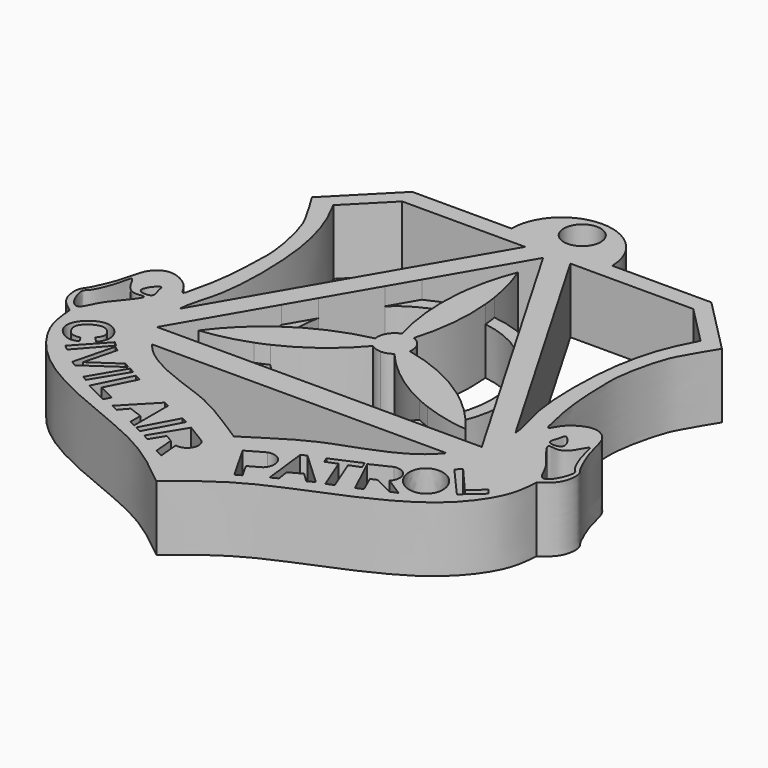
from build123d import *

# Parameters (mm, degrees)
F0_R     = 1.5875
F1_DEPTH = 5.588
F2_DEPTH = 4.064
F3_DEPTH = 3.175


# Not quite as in the source:
# - a feature names something its author has since deleted; it is built from what else it names


with BuildPart() as f1:
    # F0 (on Top) → F1 (new body)
    with BuildSketch(Plane.XY):
        with BuildLine():
            ThreePointArc((1.738595906, 17.4896921962), (-2.5962884327, 21.824576535), (-6.9311727715, 17.4896921962))
            Line((-6.9311727715, 17.4896921962), (-15.476684086, 17.4896921962))
            Line((-15.476684086, 17.4896921962), (-20.2500969172, 12.6594556496))
            add(Edge.make_bspline(
                [(-22.6898547262, -10.3722466156), (-23.0970195829, -10.0682558569), (-23.862899119, -9.4964474176), (-24.2116889935, -8.3793859815), (-24.1797927192, -7.4833620854), (-23.738938243, -7.0124281569), (-23.2773297932, -5.9756059833), (-22.8294147231, -4.8854228515), (-22.4842865284, -3.5101260949), (-22.2879650606, -2.7714005659), (-21.9081479252, -2.2626732598), (-21.271972846, -1.8143509905), (-20.3511303126, -1.7956869786), (-19.3559115764, -2.3311813439), (-18.720531189, -2.9569361713), (-18.2911432737, -3.9859192577), (-17.9733302285, -2.4199718419), (-17.4938217649, -0.258092059), (-17.3537315193, 2.707514965), (-17.2521862787, 5.0646604239), (-17.917211776, 8.1859371777), (-18.5482369005, 9.8853578959), (-19.692680388, 11.7416582003), (-20.0868858944, 12.3907254406), (-20.2500969172, 12.6594556496)],
                knots=[0, 0, 0, 0, 0.0480827662, 0.0904439714, 0.126688888, 0.1578769623, 0.1996629909, 0.244212497, 0.2916151482, 0.3262361378, 0.3571804574, 0.3915040257, 0.4288764076, 0.4706624253, 0.5103147505, 0.5426193777, 0.5825583957, 0.6451095501, 0.7133572635, 0.7758419326, 0.8458928164, 0.9011071458, 0.959055864, 1, 1, 1, 1], degree=3))
            add(Edge.make_bspline(
                [(-2.5962884327, -26.1529348791), (-3.3769549013, -25.509416408), (-4.9803315106, -24.1877220537), (-7.8461594134, -22.3308731385), (-12.0547247491, -20.6465778064), (-16.3768178003, -18.799451716), (-20.0336907945, -16.49456596), (-22.4832928257, -13.0808956511), (-22.6260637565, -11.2087384767), (-22.6898547262, -10.3722466156)],
                knots=[0, 0, 0, 0, 0.1283905799, 0.2636957792, 0.4203835822, 0.5806441644, 0.7340153977, 0.8811563698, 1, 1, 1, 1], degree=3))
            add(Edge.make_bspline(
                [(-2.5962884327, -26.1529348791), (-1.8156219642, -25.509416408), (-0.2122453549, -24.1877220537), (2.6535825479, -22.3308731385), (6.8621478837, -20.6465778064), (11.1842409349, -18.799451716), (14.841113929, -16.49456596), (17.2907159602, -13.0808956511), (17.433486891, -11.2087384767), (17.4972778607, -10.3722466156)],
                knots=[0, 0, 0, 0, 0.1283905799, 0.2636957792, 0.4203835822, 0.5806441644, 0.7340153977, 0.8811563698, 1, 1, 1, 1], degree=3))
            add(Edge.make_bspline(
                [(17.4972778607, -10.3722466156), (17.9044427174, -10.0682558569), (18.6703222535, -9.4964474176), (19.0191121281, -8.3793859815), (18.9872158537, -7.4833620854), (18.5463613775, -7.0124281569), (18.0847529277, -5.9756059833), (17.6368378576, -4.8854228515), (17.2917096629, -3.5101260949), (17.0953881952, -2.7714005659), (16.7155710597, -2.2626732598), (16.0793959805, -1.8143509905), (15.1585534472, -1.7956869786), (14.163334711, -2.3311813439), (13.5279543235, -2.9569361713), (13.0985664083, -3.9859192577), (12.780753363, -2.4199718419), (12.3012448994, -0.258092059), (12.1611546538, 2.707514965), (12.0596094132, 5.0646604239), (12.7246349105, 8.1859371777), (13.355660035, 9.8853578959), (14.5001035226, 11.7416582003), (14.8943090289, 12.3907254406), (15.0575200517, 12.6594556496)],
                knots=[0, 0, 0, 0, 0.0480827662, 0.0904439714, 0.126688888, 0.1578769623, 0.1996629909, 0.244212497, 0.2916151482, 0.3262361378, 0.3571804574, 0.3915040257, 0.4288764076, 0.4706624253, 0.5103147505, 0.5426193777, 0.5825583957, 0.6451095501, 0.7133572635, 0.7758419326, 0.8458928164, 0.9011071458, 0.959055864, 1, 1, 1, 1], degree=3))
            Line((15.0575200517, 12.6594556496), (10.2841072205, 17.4896921962))
            Line((10.2841072205, 17.4896921962), (1.738595906, 17.4896921962))
        make_face()
        Polygon((-17.8642552346, -16.1066018045), (-16.9762261212, -12.5996377319), (-16.5397357196, -12.9157155752), (-17.2622017562, -15.7002154738), (-14.9141903967, -14.089721255), (-14.4475987181, -14.3606457859), (-17.4127146602, -16.407629475), align=None, mode=Mode.SUBTRACT)
        Polygon((-15.9211166715, -17.3533935501), (-14.2067773268, -14.4359013066), (-13.7401847169, -14.7218769416), (-15.5081700509, -17.6064894405), align=None, mode=Mode.SUBTRACT)
        Polygon((-14.7967901412, -18.0994002604), (-13.2585410029, -15.0078516454), (-12.7166928723, -15.278775245), (-13.977994685, -17.801383206), (-12.5511270844, -18.51481578), (-12.8340924241, -19.0807474322), align=None, mode=Mode.SUBTRACT)
        with BuildLine():
            Line((-7.37993652, -21.467037499), (-5.6344987825, -18.6040941626))
            Line((-5.6344987825, -18.6040941626), (-3.8670410245, -19.6816521537))
            ThreePointArc((-3.8670410245, -19.6816521537), (-3.764117873, -20.8257670053), (-4.8256372102, -21.264821291))
            Line((-4.8256372102, -21.264821291), (-4.6681218682, -23.0358021975))
            Line((-4.6681218682, -23.0358021975), (-5.3577828221, -22.6909723133))
            Line((-5.3577828221, -22.6909723133), (-5.5061231892, -20.9627524731))
            Line((-5.5061231892, -20.9627524731), (-6.1475215606, -20.5717140239))
            Line((-6.1475215606, -20.5717140239), (-6.8794107919, -21.7721907597))
            Line((-6.8794107919, -21.7721907597), (-7.37993652, -21.467037499))
        make_face(mode=Mode.SUBTRACT)
        Polygon((-11.7684574798, -19.4329470396), (-9.2849843204, -16.8591663241), (-8.8304335127, -17.1150397509), (-8.8304335127, -20.7514461295), (-9.3602407724, -20.486542955), (-9.3602407724, -19.4178968668), (-10.5342464522, -18.9814064652), (-11.1784443342, -19.7279531053), align=None, mode=Mode.SUBTRACT)
        Polygon((-8.5421427919, -20.8859350641), (-6.9435769692, -17.9123040289), (-6.4029168751, -18.1826336113), (-7.9972250387, -21.1583934724), align=None, mode=Mode.SUBTRACT)
        with BuildLine():
            Line((-18.4221062809, -12.8449834883), (-18.8736468554, -12.3934429139))
            add(Edge.make_bspline(
                [(-19.6262151003, -13.0210751668), (-19.8367266487, -13.0430759324), (-20.3227133654, -13.1137191828), (-20.8027190675, -12.6674579998), (-21.1008981102, -11.9005360544), (-20.5338553761, -11.2320232518), (-19.6483014218, -10.7265798158), (-18.8566799506, -10.9897330227), (-18.4070316189, -11.7820741099), (-18.7210894211, -12.193564562), (-18.8736468554, -12.3934429139)],
                knots=[0, 0, 0, 0, 0.1176639127, 0.2306398841, 0.3539001056, 0.4832941963, 0.6263662227, 0.7518807406, 0.8786495407, 1, 1, 1, 1], degree=3))
            Line((-19.6262151003, -13.0210751668), (-19.3552915007, -13.4771401063))
            add(Edge.make_bspline(
                [(-19.3552915007, -13.4771401063), (-19.6647479685, -13.6277405765), (-20.2558959615, -13.7459268657), (-21.4140601271, -12.9898777242), (-21.7138181634, -11.531227757), (-20.0020523703, -10.0337422831), (-18.4976057776, -10.5493501512), (-17.8424780807, -11.8252496322), (-18.1724769863, -12.5210379384), (-18.4221062809, -12.8449834883)],
                knots=[0, 0, 0, 0, 0.1194322555, 0.2593120389, 0.401976621, 0.5782160681, 0.7265712091, 0.8676998255, 1, 1, 1, 1], degree=3))
        make_face(mode=Mode.SUBTRACT)
        Polygon((-19.6901927204, -14.5726281785), (-17.4127146602, -12.1029438451), (-17.0364305377, -12.4340727925), (-19.2552052424, -14.9554159103), align=None, mode=Mode.SUBTRACT)
        with BuildLine():
            add(Edge.make_bspline(
                [(-22.2999965351, -4.1639455594), (-22.1639318726, -4.1828168323), (-21.7194415576, -5.282103379), (-20.8572790048, -5.8501067699), (-19.5835447922, -5.4389447995), (-20.9052955663, -7.0779233036), (-21.9130983435, -8.2734402986), (-22.4890245815, -9.8966926591), (-23.4408419776, -9.1820975684), (-23.9767448866, -7.5276575791), (-23.4119779874, -7.3423168433), (-22.5552081146, -5.3265047979), (-22.4311477981, -4.1457557427), (-22.2999965351, -4.1639455594)],
                knots=[0, 0, 0, 0, 0.0883353731, 0.1758724355, 0.2462255334, 0.3448161859, 0.4603143006, 0.5549763071, 0.6307679108, 0.734848778, 0.7893482102, 0.9148544851, 1, 1, 1, 1], degree=3))
        make_face(mode=Mode.SUBTRACT)
        with BuildLine():
            add(Edge.make_bspline(
                [(-19.8393442792, -4.3678420189), (-19.7555659682, -4.7033214852), (-19.3308745145, -5.4325501492), (-21.474675776, -5.3829622431), (-19.8854959132, -3.4280208948), (-19.9054119199, -4.1032826531), (-19.8393442792, -4.3678420189)],
                knots=[0, 0, 0, 0, 0.2397998485, 0.5036254155, 0.8108936546, 1, 1, 1, 1], degree=3))
        make_face(mode=Mode.SUBTRACT)
        with BuildLine():
            Line((1.4085588329, -21.8684608151), (0.9114956483, -22.1504680812))
            Line((0.9114956483, -22.1504680812), (-0.8477756055, -19.0495941788))
            Line((-0.8477756055, -19.0495941788), (0.6198497044, -18.2169414814))
            ThreePointArc((0.6198497044, -18.2169414814), (1.9215311054, -18.7052821537), (1.7703687569, -20.0873100211))
            Line((1.7703687569, -20.0873100211), (0.7321975794, -20.6763132397))
            Line((0.7321975794, -20.6763132397), (1.4085588329, -21.8684608151))
        make_face(mode=Mode.SUBTRACT)
        Polygon((3.0251524877, -20.9860596806), (2.5695136283, -17.1257872134), (3.0124958139, -16.8979670852), (5.860236939, -19.5558592677), (5.3033456206, -19.8849327862), (4.4933212921, -19.100220874), (3.4428210929, -19.6697693318), (3.5947004799, -20.6949561834), align=None, mode=Mode.SUBTRACT)
        Polygon((4.4553512707, -16.8979670852), (4.2655020952, -16.4170153439), (6.7074126392, -15.3441904525), (6.9369611313, -15.9257138997), (6.0251991727, -16.2856195643), (7.1409758349, -19.1122566943), (6.5159392383, -19.3589814118), (5.3976596864, -16.5260036211), align=None, mode=Mode.SUBTRACT)
        with BuildLine():
            Line((8.4675019607, -18.593955785), (6.923393812, -15.3538584709))
            Line((6.923393812, -15.3538584709), (8.5989612084, -14.5553462599))
            ThreePointArc((8.5989612084, -14.5553462599), (9.7586835256, -15.0510769239), (9.6065988764, -16.3031052798))
            Line((9.6065988764, -16.3031052798), (11.1975504045, -17.3254568012))
            Line((11.1975504045, -17.3254568012), (10.5811590329, -17.5687689334))
            Line((10.5811590329, -17.5687689334), (8.9304475494, -16.7119012066))
            Line((8.9304475494, -16.7119012066), (8.4149169811, -16.9410266529))
            Line((8.4149169811, -16.9410266529), (9.0370504186, -18.3408223093))
            Line((9.0370504186, -18.3408223093), (8.4675019607, -18.593955785))
        make_face(mode=Mode.SUBTRACT)
        with BuildLine():
            add(Edge.make_bspline(
                [(10.3659965098, -13.3920814842), (8.3039293696, -15.1227450253), (11.119546959, -16.3837260694), (13.9351645485, -17.6447071135), (13.1816140992, -14.6530625283), (12.42806365, -11.6614179431), (10.3659965098, -13.3920814842)],
                knots=[0, 0, 0, 2.0943951024, 2.0943951024, 4.1887902048, 4.1887902048, 6.2831853072, 6.2831853072, 6.2831853072], degree=2, weights=[1, 0.5, 1, 0.5, 1, 0.5, 1]))
        make_face(mode=Mode.SUBTRACT)
        Polygon((14.3908038735, -15.0374425575), (11.9733884931, -12.2909536585), (12.4290268868, -11.9112553075), (14.4161172211, -14.2147615552), (15.605840832, -13.1769180298), (15.9995558768, -13.6214449041), align=None, mode=Mode.SUBTRACT)
        with BuildLine():
            add(Edge.make_bspline(
                [(17.1074196696, -4.1639455594), (16.9713550071, -4.1828168323), (16.5268646921, -5.282103379), (15.6647021394, -5.8501067699), (14.3909679268, -5.4389447995), (15.7127187008, -7.0779233036), (16.7205214781, -8.2734402986), (17.296447716, -9.8966926591), (18.2482651121, -9.1820975684), (18.7841680211, -7.5276575791), (18.219401122, -7.3423168433), (17.3626312491, -5.3265047979), (17.2385709326, -4.1457557427), (17.1074196696, -4.1639455594)],
                knots=[0, 0, 0, 0, 0.0883353731, 0.1758724355, 0.2462255334, 0.3448161859, 0.4603143006, 0.5549763071, 0.6307679108, 0.734848778, 0.7893482102, 0.9148544851, 1, 1, 1, 1], degree=3))
        make_face(mode=Mode.SUBTRACT)
        with BuildLine():
            add(Edge.make_bspline(
                [(14.6467674138, -4.3678420189), (14.5629891028, -4.7033214852), (14.138297649, -5.4325501492), (16.2820989106, -5.3829622431), (14.6929190477, -3.4280208948), (14.7128350544, -4.1032826531), (14.6467674138, -4.3678420189)],
                knots=[0, 0, 0, 0, 0.2397998485, 0.5036254155, 0.8108936546, 1, 1, 1, 1], degree=3))
        make_face(mode=Mode.SUBTRACT)
        with BuildLine():
            Line((-4.5437468216, 15.97869955), (-17.0728166451, -5.6040512927))
            add(Edge.make_bspline(
                [(-18.4107146599, 12.6594142163), (-18.0569607759, 11.9851124211), (-17.2122560225, 10.3749931899), (-15.9239924308, 5.9993052571), (-15.9036281511, -1.6740455136), (-16.8864107291, -4.1262955393), (-17.0494429292, -5.3143349294), (-17.0728166451, -5.6040512927)],
                knots=[0, 0, 0, 0, 0.0808340305, 0.1930180639, 0.3369454066, 0.4287723959, 0.4590184966, 0.4590184966, 0.4590184966, 0.4590184966], degree=3))
            Line((-18.4107146599, 12.6594142163), (-15.1304779574, 15.97869955))
            Line((-15.1304779574, 15.97869955), (-4.5437468216, 15.97869955))
        make_face(mode=Mode.SUBTRACT)
        with Locations((-2.5962884327, 19.6944624186)):
            Circle(F0_R, mode=Mode.SUBTRACT)
        with BuildLine():
            add(Edge.make_bspline(
                [(10.0973419707, -10.7784895471), (9.7674807888, -11.1849337214), (7.9960155748, -12.9796550021), (2.9873140765, -14.4563732252), (0.4737445345, -15.8470104966), (-1.5423590099, -17.1389273944), (-2.5962884327, -17.8142841905)],
                knots=[0.6433469653, 0.6433469653, 0.6433469653, 0.6433469653, 0.6805727904, 0.8122831254, 0.9018699521, 1, 1, 1, 1], degree=3))
            add(Edge.make_bspline(
                [(-15.2899188362, -10.7784895471), (-14.9600576543, -11.1849337214), (-13.1885924403, -12.9796550021), (-8.179890942, -14.4563732252), (-5.6663214, -15.8470104966), (-3.6502178555, -17.1389273944), (-2.5962884327, -17.8142841905)],
                knots=[0.6433469653, 0.6433469653, 0.6433469653, 0.6433469653, 0.6805727904, 0.8122831254, 0.9018699521, 1, 1, 1, 1], degree=3))
            add(Edge.make_bspline(
                [(-16.5762994438, -8.6002144963), (-16.3015036385, -9.240777885), (-15.8987416853, -10.0283179179), (-15.2899188362, -10.7784895471)],
                knots=[0.5746394784, 0.5746394784, 0.5746394784, 0.5746394784, 0.6433469653, 0.6433469653, 0.6433469653, 0.6433469653], degree=3))
            Line((-16.5762994438, -8.6002144963), (-12.0692629629, -0.8363304429))
            Line((-12.0692629629, -0.8363304429), (-10.7320598082, 1.4671544065))
            Line((-10.7320598082, 1.4671544065), (-8.3266215781, 5.6107959312))
            Line((-8.3266215781, 5.6107959312), (-6.9894184233, 7.9142807806))
            Line((-6.9894184233, 7.9142807806), (-2.5962884327, 15.4819479212))
            Line((-2.5962884327, 15.4819479212), (1.7968415578, 7.9142807806))
            Line((1.7968415578, 7.9142807806), (3.1340447126, 5.6107959312))
            Line((3.1340447126, 5.6107959312), (5.5394829427, 1.4671544065))
            Line((5.5394829427, 1.4671544065), (6.8766860975, -0.8363304429))
            Line((6.8766860975, -0.8363304429), (11.3837225784, -8.6002144963))
            add(Edge.make_bspline(
                [(11.3837225784, -8.6002144963), (11.108926773, -9.240777885), (10.7061648198, -10.0283179179), (10.0973419707, -10.7784895471)],
                knots=[0.5746394784, 0.5746394784, 0.5746394784, 0.5746394784, 0.6433469653, 0.6433469653, 0.6433469653, 0.6433469653], degree=3))
        make_face(mode=Mode.SUBTRACT)
        with BuildLine():
            add(Edge.make_bspline(
                [(13.2181377944, 12.6594142163), (12.8643839105, 11.9851124211), (12.019679157, 10.3749931899), (10.7314155654, 5.9993052571), (10.7110512856, -1.6740455136), (11.6938338637, -4.1262955393), (11.8568660637, -5.3143349294), (11.8802397797, -5.6040512927)],
                knots=[0, 0, 0, 0, 0.0808340305, 0.1930180639, 0.3369454066, 0.4287723959, 0.4590184966, 0.4590184966, 0.4590184966, 0.4590184966], degree=3))
            Line((11.8802397797, -5.6040512927), (-0.6488300439, 15.97869955))
            Line((-0.6488300439, 15.97869955), (9.937901092, 15.97869955))
            Line((9.937901092, 15.97869955), (13.2181377944, 12.6594142163))
        make_face(mode=Mode.SUBTRACT)
        with BuildLine():
            Line((-15.2899188362, -10.7784895471), (-2.5962884327, -10.7784895471))
            Line((-2.5962884327, -10.7784895471), (-2.5962884327, -8.6002144963))
            Line((-2.5962884327, -8.6002144963), (-4.6359278745, -8.6002144963))
            Line((-4.6359278745, -8.6002144963), (-7.4968658318, -8.6002144963))
            Line((-7.4968658318, -8.6002144963), (-16.5762994438, -8.6002144963))
            add(Edge.make_bspline(
                [(-16.5762994438, -8.6002144963), (-16.3015036385, -9.240777885), (-15.8987416853, -10.0283179179), (-15.2899188362, -10.7784895471)],
                knots=[0.5746394784, 0.5746394784, 0.5746394784, 0.5746394784, 0.6433469653, 0.6433469653, 0.6433469653, 0.6433469653], degree=3))
        make_face()
        with BuildLine():
            Line((-2.5962884327, -8.6002144963), (-2.5962884327, -10.7784895471))
            Line((-2.5962884327, -10.7784895471), (10.0973419707, -10.7784895471))
            add(Edge.make_bspline(
                [(11.3837225784, -8.6002144963), (11.108926773, -9.240777885), (10.7061648198, -10.0283179179), (10.0973419707, -10.7784895471)],
                knots=[0.5746394784, 0.5746394784, 0.5746394784, 0.5746394784, 0.6433469653, 0.6433469653, 0.6433469653, 0.6433469653], degree=3))
            Line((11.3837225784, -8.6002144963), (2.3042889663, -8.6002144963))
            Line((2.3042889663, -8.6002144963), (-0.556648991, -8.6002144963))
            Line((-0.556648991, -8.6002144963), (-2.5962884327, -8.6002144963))
        make_face()
    extrude(amount=F1_DEPTH)



with BuildPart() as f1b:
    # F0 (on Top) → F1, piece 2 (new body)
    with BuildSketch(Plane.XY):
        with BuildLine():
            ThreePointArc((-3.5194281199, -1.6833554323), (-3.0839086469, -1.9170687551), (-2.5962884327, -1.9978502831))
            ThreePointArc((-2.5962884327, -1.9978502831), (-2.1086682185, -1.9170687551), (-1.6731487456, -1.6833554323))
            ThreePointArc((-1.6731487456, -1.6833554323), (-1.2996969194, -1.2637563943), (-1.1051752701, -0.7367924989))
            ThreePointArc((-1.1051752701, -0.7367924989), (-1.0894459848, -0.6117102954), (-1.0841907134, -0.4857525637))
            ThreePointArc((-1.0841907134, -0.4857525637), (-1.3642345669, 0.3908789351), (-2.1006366412, 0.9428022356))
            ThreePointArc((-2.1006366412, 0.9428022356), (-2.5962884327, 1.0263451557), (-3.0919402242, 0.9428022356))
            ThreePointArc((-3.0919402242, 0.9428022356), (-3.897083714, 0.2852021361), (-4.0874015954, -0.7367924989))
            ThreePointArc((-4.0874015954, -0.7367924989), (-3.8928799461, -1.2637563943), (-3.5194281199, -1.6833554323))
        make_face()
        with BuildLine():
            ThreePointArc((-10.0793335963, -6.3050468834), (-9.5411639221, -6.0908981171), (-9.0110868051, -5.8574360381))
            ThreePointArc((-9.0110868051, -5.8574360381), (-6.037948215, -4.0694567551), (-3.5194281199, -1.6833554323))
            ThreePointArc((-3.5194281199, -1.6833554323), (-3.8928799461, -1.2637563943), (-4.0874015954, -0.7367924989))
            ThreePointArc((-4.0874015954, -0.7367924989), (-7.3817282518, -1.8136482669), (-10.3830788025, -3.5468826238))
            ThreePointArc((-10.3830788025, -3.5468826238), (-10.8444096754, -3.8938575644), (-11.2934819225, -4.2565584061))
            ThreePointArc((-11.2934819225, -4.2565584061), (-12.7839417852, -5.6678497623), (-14.0901431441, -7.25121703))
            ThreePointArc((-14.0901431441, -7.25121703), (-12.0541901869, -6.9076255218), (-10.0793335963, -6.3050468834))
        make_face()
        with BuildLine():
            ThreePointArc((-1.1051752701, -0.7367924989), (-1.2996969194, -1.2637563943), (-1.6731487456, -1.6833554323))
            ThreePointArc((-1.6731487456, -1.6833554323), (0.8453713496, -4.0694567551), (3.8185099396, -5.8574360381))
            ThreePointArc((3.8185099396, -5.8574360381), (4.3485870566, -6.0908981171), (4.8867567308, -6.3050468834))
            ThreePointArc((4.8867567308, -6.3050468834), (6.8616133214, -6.9076255218), (8.8975662787, -7.25121703))
            ThreePointArc((8.8975662787, -7.25121703), (7.5913649198, -5.6678497623), (6.100905057, -4.2565584061))
            ThreePointArc((6.100905057, -4.2565584061), (5.6518328099, -3.8938575644), (5.190501937, -3.5468826238))
            ThreePointArc((5.190501937, -3.5468826238), (2.1891513863, -1.8136482669), (-1.1051752701, -0.7367924989))
        make_face()
        with BuildLine():
            ThreePointArc((-3.7813396998, 7.796775734), (-3.7663862952, 4.3366218082), (-3.0919402242, 0.9428022356))
            ThreePointArc((-3.0919402242, 0.9428022356), (-2.5962884327, 1.0263451557), (-2.1006366412, 0.9428022356))
            ThreePointArc((-2.1006366412, 0.9428022356), (-1.4261905703, 4.3366218082), (-1.4112371657, 7.796775734))
            ThreePointArc((-1.4112371657, 7.796775734), (-1.4728293716, 8.3675449449), (-1.5525279601, 8.9360686708))
            ThreePointArc((-1.5525279601, 8.9360686708), (-1.9684242871, 10.8841323421), (-2.5962884327, 12.7745578066))
            ThreePointArc((-2.5962884327, 12.7745578066), (-3.2241525784, 10.8841323421), (-3.6400489054, 8.9360686708))
            ThreePointArc((-3.6400489054, 8.9360686708), (-3.7197474939, 8.3675449449), (-3.7813396998, 7.796775734))
        make_face()
    extrude(amount=F1_DEPTH)


with BuildPart() as f1_1:
    add(f1.part)

    add(f1b.part)  # F2 merges F1b
    # F0 (on Top) → F2 (join)
    with BuildSketch(Plane.XY):
        with BuildLine():
            Line((-6.9894184233, 7.9142807806), (-8.3266215781, 5.6107959312))
            ThreePointArc((-8.3266215781, 5.6107959312), (-6.2226174743, 7.0544304042), (-3.7813396998, 7.796775734))
            ThreePointArc((-3.7813396998, 7.796775734), (-3.7197474939, 8.3675449449), (-3.6400489054, 8.9360686708))
            ThreePointArc((-3.6400489054, 8.9360686708), (-5.3623247847, 8.5811760342), (-6.9894184233, 7.9142807806))
        make_face()
        with BuildLine():
            ThreePointArc((-1.4112371657, 7.796775734), (1.0300406088, 7.0544304042), (3.1340447126, 5.6107959312))
            Line((3.1340447126, 5.6107959312), (1.7968415578, 7.9142807806))
            ThreePointArc((1.7968415578, 7.9142807806), (0.1697479192, 8.5811760342), (-1.5525279601, 8.9360686708))
            ThreePointArc((-1.5525279601, 8.9360686708), (-1.4728293716, 8.3675449449), (-1.4112371657, 7.796775734))
        make_face()
        with BuildLine():
            ThreePointArc((6.100905057, -4.2565584061), (6.6483446751, -2.5826335811), (6.8766860975, -0.8363304429))
            Line((6.8766860975, -0.8363304429), (5.5394829427, 1.4671544065))
            ThreePointArc((5.5394829427, 1.4671544065), (5.7503956374, -1.0666884809), (5.190501937, -3.5468826238))
            ThreePointArc((5.190501937, -3.5468826238), (5.6518328099, -3.8938575644), (6.100905057, -4.2565584061))
        make_face()
        with BuildLine():
            ThreePointArc((3.8185099396, -5.8574360381), (1.8478186886, -7.5747957574), (-0.556648991, -8.6002144963))
            Line((-0.556648991, -8.6002144963), (2.3042889663, -8.6002144963))
            ThreePointArc((2.3042889663, -8.6002144963), (3.7009709343, -7.5712783567), (4.8867567308, -6.3050468834))
            ThreePointArc((4.8867567308, -6.3050468834), (4.3485870566, -6.0908981171), (3.8185099396, -5.8574360381))
        make_face()
        with BuildLine():
            Line((-7.4968658318, -8.6002144963), (-4.6359278745, -8.6002144963))
            ThreePointArc((-4.6359278745, -8.6002144963), (-7.040395554, -7.5747957574), (-9.0110868051, -5.8574360381))
            ThreePointArc((-9.0110868051, -5.8574360381), (-9.5411639221, -6.0908981171), (-10.0793335963, -6.3050468834))
            ThreePointArc((-10.0793335963, -6.3050468834), (-8.8935477998, -7.5712783567), (-7.4968658318, -8.6002144963))
        make_face()
        with BuildLine():
            Line((-10.7320598082, 1.4671544065), (-12.0692629629, -0.8363304429))
            ThreePointArc((-12.0692629629, -0.8363304429), (-11.8409215406, -2.5826335811), (-11.2934819225, -4.2565584061))
            ThreePointArc((-11.2934819225, -4.2565584061), (-10.8444096754, -3.8938575644), (-10.3830788025, -3.5468826238))
            ThreePointArc((-10.3830788025, -3.5468826238), (-10.9429725029, -1.0666884809), (-10.7320598082, 1.4671544065))
        make_face()
    extrude(amount=F2_DEPTH)

    # F0 (on Top) → F3 (join)
    with BuildSketch(Plane.XY):
        with BuildLine():
            ThreePointArc((1.738595906, 17.4896921962), (-2.5962884327, 21.824576535), (-6.9311727715, 17.4896921962))
            Line((-6.9311727715, 17.4896921962), (-15.476684086, 17.4896921962))
            Line((-15.476684086, 17.4896921962), (-20.2500969172, 12.6594556496))
            add(Edge.make_bspline(
                [(-22.6898547262, -10.3722466156), (-23.0970195829, -10.0682558569), (-23.862899119, -9.4964474176), (-24.2116889935, -8.3793859815), (-24.1797927192, -7.4833620854), (-23.738938243, -7.0124281569), (-23.2773297932, -5.9756059833), (-22.8294147231, -4.8854228515), (-22.4842865284, -3.5101260949), (-22.2879650606, -2.7714005659), (-21.9081479252, -2.2626732598), (-21.271972846, -1.8143509905), (-20.3511303126, -1.7956869786), (-19.3559115764, -2.3311813439), (-18.720531189, -2.9569361713), (-18.2911432737, -3.9859192577), (-17.9733302285, -2.4199718419), (-17.4938217649, -0.258092059), (-17.3537315193, 2.707514965), (-17.2521862787, 5.0646604239), (-17.917211776, 8.1859371777), (-18.5482369005, 9.8853578959), (-19.692680388, 11.7416582003), (-20.0868858944, 12.3907254406), (-20.2500969172, 12.6594556496)],
                knots=[0, 0, 0, 0, 0.0480827662, 0.0904439714, 0.126688888, 0.1578769623, 0.1996629909, 0.244212497, 0.2916151482, 0.3262361378, 0.3571804574, 0.3915040257, 0.4288764076, 0.4706624253, 0.5103147505, 0.5426193777, 0.5825583957, 0.6451095501, 0.7133572635, 0.7758419326, 0.8458928164, 0.9011071458, 0.959055864, 1, 1, 1, 1], degree=3))
            add(Edge.make_bspline(
                [(-2.5962884327, -26.1529348791), (-3.3769549013, -25.509416408), (-4.9803315106, -24.1877220537), (-7.8461594134, -22.3308731385), (-12.0547247491, -20.6465778064), (-16.3768178003, -18.799451716), (-20.0336907945, -16.49456596), (-22.4832928257, -13.0808956511), (-22.6260637565, -11.2087384767), (-22.6898547262, -10.3722466156)],
                knots=[0, 0, 0, 0, 0.1283905799, 0.2636957792, 0.4203835822, 0.5806441644, 0.7340153977, 0.8811563698, 1, 1, 1, 1], degree=3))
            add(Edge.make_bspline(
                [(-2.5962884327, -26.1529348791), (-1.8156219642, -25.509416408), (-0.2122453549, -24.1877220537), (2.6535825479, -22.3308731385), (6.8621478837, -20.6465778064), (11.1842409349, -18.799451716), (14.841113929, -16.49456596), (17.2907159602, -13.0808956511), (17.433486891, -11.2087384767), (17.4972778607, -10.3722466156)],
                knots=[0, 0, 0, 0, 0.1283905799, 0.2636957792, 0.4203835822, 0.5806441644, 0.7340153977, 0.8811563698, 1, 1, 1, 1], degree=3))
            add(Edge.make_bspline(
                [(17.4972778607, -10.3722466156), (17.9044427174, -10.0682558569), (18.6703222535, -9.4964474176), (19.0191121281, -8.3793859815), (18.9872158537, -7.4833620854), (18.5463613775, -7.0124281569), (18.0847529277, -5.9756059833), (17.6368378576, -4.8854228515), (17.2917096629, -3.5101260949), (17.0953881952, -2.7714005659), (16.7155710597, -2.2626732598), (16.0793959805, -1.8143509905), (15.1585534472, -1.7956869786), (14.163334711, -2.3311813439), (13.5279543235, -2.9569361713), (13.0985664083, -3.9859192577), (12.780753363, -2.4199718419), (12.3012448994, -0.258092059), (12.1611546538, 2.707514965), (12.0596094132, 5.0646604239), (12.7246349105, 8.1859371777), (13.355660035, 9.8853578959), (14.5001035226, 11.7416582003), (14.8943090289, 12.3907254406), (15.0575200517, 12.6594556496)],
                knots=[0, 0, 0, 0, 0.0480827662, 0.0904439714, 0.126688888, 0.1578769623, 0.1996629909, 0.244212497, 0.2916151482, 0.3262361378, 0.3571804574, 0.3915040257, 0.4288764076, 0.4706624253, 0.5103147505, 0.5426193777, 0.5825583957, 0.6451095501, 0.7133572635, 0.7758419326, 0.8458928164, 0.9011071458, 0.959055864, 1, 1, 1, 1], degree=3))
            Line((15.0575200517, 12.6594556496), (10.2841072205, 17.4896921962))
            Line((10.2841072205, 17.4896921962), (1.738595906, 17.4896921962))
        make_face()
        Polygon((-17.8642552346, -16.1066018045), (-16.9762261212, -12.5996377319), (-16.5397357196, -12.9157155752), (-17.2622017562, -15.7002154738), (-14.9141903967, -14.089721255), (-14.4475987181, -14.3606457859), (-17.4127146602, -16.407629475), align=None, mode=Mode.SUBTRACT)
        Polygon((-15.9211166715, -17.3533935501), (-14.2067773268, -14.4359013066), (-13.7401847169, -14.7218769416), (-15.5081700509, -17.6064894405), align=None, mode=Mode.SUBTRACT)
        Polygon((-14.7967901412, -18.0994002604), (-13.2585410029, -15.0078516454), (-12.7166928723, -15.278775245), (-13.977994685, -17.801383206), (-12.5511270844, -18.51481578), (-12.8340924241, -19.0807474322), align=None, mode=Mode.SUBTRACT)
        with BuildLine():
            Line((-7.37993652, -21.467037499), (-5.6344987825, -18.6040941626))
            Line((-5.6344987825, -18.6040941626), (-3.8670410245, -19.6816521537))
            ThreePointArc((-3.8670410245, -19.6816521537), (-3.764117873, -20.8257670053), (-4.8256372102, -21.264821291))
            Line((-4.8256372102, -21.264821291), (-4.6681218682, -23.0358021975))
            Line((-4.6681218682, -23.0358021975), (-5.3577828221, -22.6909723133))
            Line((-5.3577828221, -22.6909723133), (-5.5061231892, -20.9627524731))
            Line((-5.5061231892, -20.9627524731), (-6.1475215606, -20.5717140239))
            Line((-6.1475215606, -20.5717140239), (-6.8794107919, -21.7721907597))
            Line((-6.8794107919, -21.7721907597), (-7.37993652, -21.467037499))
        make_face(mode=Mode.SUBTRACT)
        Polygon((-11.7684574798, -19.4329470396), (-9.2849843204, -16.8591663241), (-8.8304335127, -17.1150397509), (-8.8304335127, -20.7514461295), (-9.3602407724, -20.486542955), (-9.3602407724, -19.4178968668), (-10.5342464522, -18.9814064652), (-11.1784443342, -19.7279531053), align=None, mode=Mode.SUBTRACT)
        Polygon((-8.5421427919, -20.8859350641), (-6.9435769692, -17.9123040289), (-6.4029168751, -18.1826336113), (-7.9972250387, -21.1583934724), align=None, mode=Mode.SUBTRACT)
        with BuildLine():
            Line((-18.4221062809, -12.8449834883), (-18.8736468554, -12.3934429139))
            add(Edge.make_bspline(
                [(-19.6262151003, -13.0210751668), (-19.8367266487, -13.0430759324), (-20.3227133654, -13.1137191828), (-20.8027190675, -12.6674579998), (-21.1008981102, -11.9005360544), (-20.5338553761, -11.2320232518), (-19.6483014218, -10.7265798158), (-18.8566799506, -10.9897330227), (-18.4070316189, -11.7820741099), (-18.7210894211, -12.193564562), (-18.8736468554, -12.3934429139)],
                knots=[0, 0, 0, 0, 0.1176639127, 0.2306398841, 0.3539001056, 0.4832941963, 0.6263662227, 0.7518807406, 0.8786495407, 1, 1, 1, 1], degree=3))
            Line((-19.6262151003, -13.0210751668), (-19.3552915007, -13.4771401063))
            add(Edge.make_bspline(
                [(-19.3552915007, -13.4771401063), (-19.6647479685, -13.6277405765), (-20.2558959615, -13.7459268657), (-21.4140601271, -12.9898777242), (-21.7138181634, -11.531227757), (-20.0020523703, -10.0337422831), (-18.4976057776, -10.5493501512), (-17.8424780807, -11.8252496322), (-18.1724769863, -12.5210379384), (-18.4221062809, -12.8449834883)],
                knots=[0, 0, 0, 0, 0.1194322555, 0.2593120389, 0.401976621, 0.5782160681, 0.7265712091, 0.8676998255, 1, 1, 1, 1], degree=3))
        make_face(mode=Mode.SUBTRACT)
        Polygon((-19.6901927204, -14.5726281785), (-17.4127146602, -12.1029438451), (-17.0364305377, -12.4340727925), (-19.2552052424, -14.9554159103), align=None, mode=Mode.SUBTRACT)
        with BuildLine():
            add(Edge.make_bspline(
                [(-22.2999965351, -4.1639455594), (-22.1639318726, -4.1828168323), (-21.7194415576, -5.282103379), (-20.8572790048, -5.8501067699), (-19.5835447922, -5.4389447995), (-20.9052955663, -7.0779233036), (-21.9130983435, -8.2734402986), (-22.4890245815, -9.8966926591), (-23.4408419776, -9.1820975684), (-23.9767448866, -7.5276575791), (-23.4119779874, -7.3423168433), (-22.5552081146, -5.3265047979), (-22.4311477981, -4.1457557427), (-22.2999965351, -4.1639455594)],
                knots=[0, 0, 0, 0, 0.0883353731, 0.1758724355, 0.2462255334, 0.3448161859, 0.4603143006, 0.5549763071, 0.6307679108, 0.734848778, 0.7893482102, 0.9148544851, 1, 1, 1, 1], degree=3))
        make_face(mode=Mode.SUBTRACT)
        with BuildLine():
            add(Edge.make_bspline(
                [(-19.8393442792, -4.3678420189), (-19.7555659682, -4.7033214852), (-19.3308745145, -5.4325501492), (-21.474675776, -5.3829622431), (-19.8854959132, -3.4280208948), (-19.9054119199, -4.1032826531), (-19.8393442792, -4.3678420189)],
                knots=[0, 0, 0, 0, 0.2397998485, 0.5036254155, 0.8108936546, 1, 1, 1, 1], degree=3))
        make_face(mode=Mode.SUBTRACT)
        with BuildLine():
            Line((1.4085588329, -21.8684608151), (0.9114956483, -22.1504680812))
            Line((0.9114956483, -22.1504680812), (-0.8477756055, -19.0495941788))
            Line((-0.8477756055, -19.0495941788), (0.6198497044, -18.2169414814))
            ThreePointArc((0.6198497044, -18.2169414814), (1.9215311054, -18.7052821537), (1.7703687569, -20.0873100211))
            Line((1.7703687569, -20.0873100211), (0.7321975794, -20.6763132397))
            Line((0.7321975794, -20.6763132397), (1.4085588329, -21.8684608151))
        make_face(mode=Mode.SUBTRACT)
        Polygon((3.0251524877, -20.9860596806), (2.5695136283, -17.1257872134), (3.0124958139, -16.8979670852), (5.860236939, -19.5558592677), (5.3033456206, -19.8849327862), (4.4933212921, -19.100220874), (3.4428210929, -19.6697693318), (3.5947004799, -20.6949561834), align=None, mode=Mode.SUBTRACT)
        Polygon((4.4553512707, -16.8979670852), (4.2655020952, -16.4170153439), (6.7074126392, -15.3441904525), (6.9369611313, -15.9257138997), (6.0251991727, -16.2856195643), (7.1409758349, -19.1122566943), (6.5159392383, -19.3589814118), (5.3976596864, -16.5260036211), align=None, mode=Mode.SUBTRACT)
        with BuildLine():
            Line((8.4675019607, -18.593955785), (6.923393812, -15.3538584709))
            Line((6.923393812, -15.3538584709), (8.5989612084, -14.5553462599))
            ThreePointArc((8.5989612084, -14.5553462599), (9.7586835256, -15.0510769239), (9.6065988764, -16.3031052798))
            Line((9.6065988764, -16.3031052798), (11.1975504045, -17.3254568012))
            Line((11.1975504045, -17.3254568012), (10.5811590329, -17.5687689334))
            Line((10.5811590329, -17.5687689334), (8.9304475494, -16.7119012066))
            Line((8.9304475494, -16.7119012066), (8.4149169811, -16.9410266529))
            Line((8.4149169811, -16.9410266529), (9.0370504186, -18.3408223093))
            Line((9.0370504186, -18.3408223093), (8.4675019607, -18.593955785))
        make_face(mode=Mode.SUBTRACT)
        with BuildLine():
            add(Edge.make_bspline(
                [(10.3659965098, -13.3920814842), (8.3039293696, -15.1227450253), (11.119546959, -16.3837260694), (13.9351645485, -17.6447071135), (13.1816140992, -14.6530625283), (12.42806365, -11.6614179431), (10.3659965098, -13.3920814842)],
                knots=[0, 0, 0, 2.0943951024, 2.0943951024, 4.1887902048, 4.1887902048, 6.2831853072, 6.2831853072, 6.2831853072], degree=2, weights=[1, 0.5, 1, 0.5, 1, 0.5, 1]))
        make_face(mode=Mode.SUBTRACT)
        Polygon((14.3908038735, -15.0374425575), (11.9733884931, -12.2909536585), (12.4290268868, -11.9112553075), (14.4161172211, -14.2147615552), (15.605840832, -13.1769180298), (15.9995558768, -13.6214449041), align=None, mode=Mode.SUBTRACT)
        with BuildLine():
            add(Edge.make_bspline(
                [(17.1074196696, -4.1639455594), (16.9713550071, -4.1828168323), (16.5268646921, -5.282103379), (15.6647021394, -5.8501067699), (14.3909679268, -5.4389447995), (15.7127187008, -7.0779233036), (16.7205214781, -8.2734402986), (17.296447716, -9.8966926591), (18.2482651121, -9.1820975684), (18.7841680211, -7.5276575791), (18.219401122, -7.3423168433), (17.3626312491, -5.3265047979), (17.2385709326, -4.1457557427), (17.1074196696, -4.1639455594)],
                knots=[0, 0, 0, 0, 0.0883353731, 0.1758724355, 0.2462255334, 0.3448161859, 0.4603143006, 0.5549763071, 0.6307679108, 0.734848778, 0.7893482102, 0.9148544851, 1, 1, 1, 1], degree=3))
        make_face(mode=Mode.SUBTRACT)
        with BuildLine():
            add(Edge.make_bspline(
                [(14.6467674138, -4.3678420189), (14.5629891028, -4.7033214852), (14.138297649, -5.4325501492), (16.2820989106, -5.3829622431), (14.6929190477, -3.4280208948), (14.7128350544, -4.1032826531), (14.6467674138, -4.3678420189)],
                knots=[0, 0, 0, 0, 0.2397998485, 0.5036254155, 0.8108936546, 1, 1, 1, 1], degree=3))
        make_face(mode=Mode.SUBTRACT)
        with BuildLine():
            Line((-4.5437468216, 15.97869955), (-17.0728166451, -5.6040512927))
            add(Edge.make_bspline(
                [(-18.4107146599, 12.6594142163), (-18.0569607759, 11.9851124211), (-17.2122560225, 10.3749931899), (-15.9239924308, 5.9993052571), (-15.9036281511, -1.6740455136), (-16.8864107291, -4.1262955393), (-17.0494429292, -5.3143349294), (-17.0728166451, -5.6040512927)],
                knots=[0, 0, 0, 0, 0.0808340305, 0.1930180639, 0.3369454066, 0.4287723959, 0.4590184966, 0.4590184966, 0.4590184966, 0.4590184966], degree=3))
            Line((-18.4107146599, 12.6594142163), (-15.1304779574, 15.97869955))
            Line((-15.1304779574, 15.97869955), (-4.5437468216, 15.97869955))
        make_face(mode=Mode.SUBTRACT)
        with Locations((-2.5962884327, 19.6944624186)):
            Circle(F0_R, mode=Mode.SUBTRACT)
        with BuildLine():
            add(Edge.make_bspline(
                [(10.0973419707, -10.7784895471), (9.7674807888, -11.1849337214), (7.9960155748, -12.9796550021), (2.9873140765, -14.4563732252), (0.4737445345, -15.8470104966), (-1.5423590099, -17.1389273944), (-2.5962884327, -17.8142841905)],
                knots=[0.6433469653, 0.6433469653, 0.6433469653, 0.6433469653, 0.6805727904, 0.8122831254, 0.9018699521, 1, 1, 1, 1], degree=3))
            add(Edge.make_bspline(
                [(-15.2899188362, -10.7784895471), (-14.9600576543, -11.1849337214), (-13.1885924403, -12.9796550021), (-8.179890942, -14.4563732252), (-5.6663214, -15.8470104966), (-3.6502178555, -17.1389273944), (-2.5962884327, -17.8142841905)],
                knots=[0.6433469653, 0.6433469653, 0.6433469653, 0.6433469653, 0.6805727904, 0.8122831254, 0.9018699521, 1, 1, 1, 1], degree=3))
            add(Edge.make_bspline(
                [(-16.5762994438, -8.6002144963), (-16.3015036385, -9.240777885), (-15.8987416853, -10.0283179179), (-15.2899188362, -10.7784895471)],
                knots=[0.5746394784, 0.5746394784, 0.5746394784, 0.5746394784, 0.6433469653, 0.6433469653, 0.6433469653, 0.6433469653], degree=3))
            Line((-16.5762994438, -8.6002144963), (-12.0692629629, -0.8363304429))
            Line((-12.0692629629, -0.8363304429), (-10.7320598082, 1.4671544065))
            Line((-10.7320598082, 1.4671544065), (-8.3266215781, 5.6107959312))
            Line((-8.3266215781, 5.6107959312), (-6.9894184233, 7.9142807806))
            Line((-6.9894184233, 7.9142807806), (-2.5962884327, 15.4819479212))
            Line((-2.5962884327, 15.4819479212), (1.7968415578, 7.9142807806))
            Line((1.7968415578, 7.9142807806), (3.1340447126, 5.6107959312))
            Line((3.1340447126, 5.6107959312), (5.5394829427, 1.4671544065))
            Line((5.5394829427, 1.4671544065), (6.8766860975, -0.8363304429))
            Line((6.8766860975, -0.8363304429), (11.3837225784, -8.6002144963))
            add(Edge.make_bspline(
                [(11.3837225784, -8.6002144963), (11.108926773, -9.240777885), (10.7061648198, -10.0283179179), (10.0973419707, -10.7784895471)],
                knots=[0.5746394784, 0.5746394784, 0.5746394784, 0.5746394784, 0.6433469653, 0.6433469653, 0.6433469653, 0.6433469653], degree=3))
        make_face(mode=Mode.SUBTRACT)
        with BuildLine():
            add(Edge.make_bspline(
                [(13.2181377944, 12.6594142163), (12.8643839105, 11.9851124211), (12.019679157, 10.3749931899), (10.7314155654, 5.9993052571), (10.7110512856, -1.6740455136), (11.6938338637, -4.1262955393), (11.8568660637, -5.3143349294), (11.8802397797, -5.6040512927)],
                knots=[0, 0, 0, 0, 0.0808340305, 0.1930180639, 0.3369454066, 0.4287723959, 0.4590184966, 0.4590184966, 0.4590184966, 0.4590184966], degree=3))
            Line((11.8802397797, -5.6040512927), (-0.6488300439, 15.97869955))
            Line((-0.6488300439, 15.97869955), (9.937901092, 15.97869955))
            Line((9.937901092, 15.97869955), (13.2181377944, 12.6594142163))
        make_face(mode=Mode.SUBTRACT)
    extrude(amount=F3_DEPTH)


solid = f1_1.part
